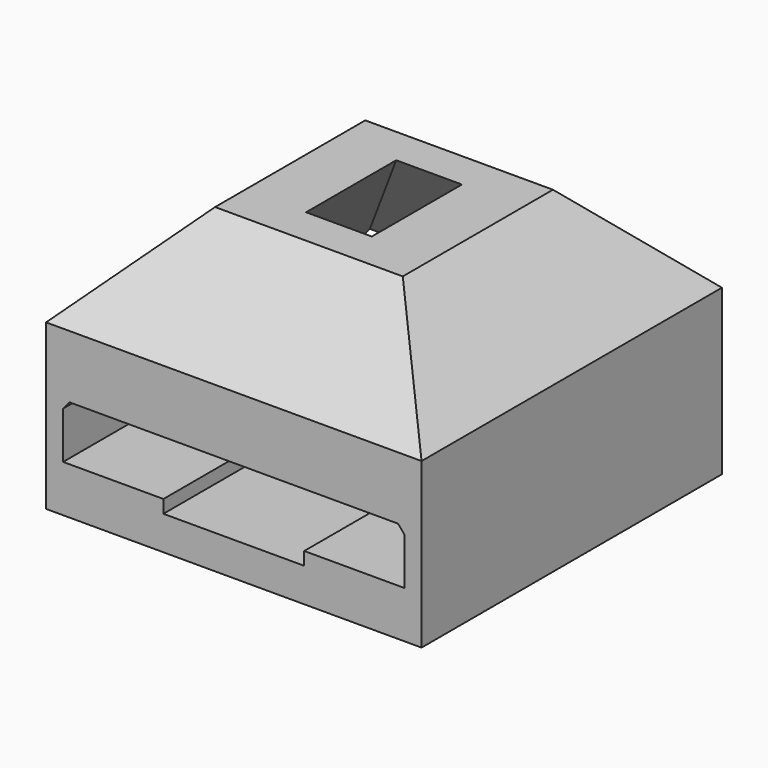
from build123d import *

# Parameters (mm, degrees)
F0_W     = 80
F0_H     = 80
F1_DEPTH = 55
F2_SIZE2 = 20
F2_SIZE  = 20
F3_W     = 14
F3_H     = 24
F4_DEPTH = 35
F4_TAPER = -40
F5_W     = 15
F5_H     = 2.5
F5_H_2   = 5.2806121111
F6_DEPTH = 50
F7_DEPTH = 10
F8_DEPTH = 5


# Not quite as in the source:
# - a feature names something its author has since deleted; it is built from what else it names


with BuildPart() as f1:
    # F0 (on Top) → F1 (new body)
    with BuildSketch(Plane.XY):
        with Locations((3.4524537623, -3.0448271871)):
            Rectangle(F0_W, F0_H)
    extrude(amount=F1_DEPTH)

    # F2
    f2_edges = [f1.edges().sort_by_distance(p)[0] for p in [
        (43.452454, -3.044827, 55),
        (3.452454, 36.955173, 55),
        (-36.547546, -3.044827, 55),
        (3.452454, -43.044827, 55),
    ]]
    chamfer(f2_edges, length=F2_SIZE, length2=F2_SIZE2)

    # F3 (on face) → F4 (cut)
    with BuildSketch(Plane.XY.offset(55)):
        with Locations((3.4524537623, -3.0448271871)):
            Rectangle(F3_W, F3_H)
    extrude(amount=-F4_DEPTH, taper=F4_TAPER, mode=Mode.SUBTRACT)

    # F5 (on face) → F6 (cut)
    with BuildSketch(Plane.XZ.offset(43.0448271871)):
        with Locations((10.9524537623, 18.75)):
            Rectangle(F5_W, F5_H)
        with Locations((-4.0475462377, 18.75)):
            Rectangle(F5_W, F5_H)
        with Locations((-4.0475462377, 14.8596939445)):
            Rectangle(F5_W, F5_H_2)
        with Locations((10.9524537623, 14.8596939445)):
            Rectangle(F5_W, F5_H_2)
    extrude(amount=-F6_DEPTH, mode=Mode.SUBTRACT)

    # F7 (cut): a face of the model
    f7_faces = [f1.faces().sort_by_distance(p)[0] for p in [
        (3.4524537623, 35.8739389153, 20),
    ]]
    extrude(f7_faces, amount=-F7_DEPTH, mode=Mode.SUBTRACT)

    # F8 (cut): a face of the model
    f8_faces = [f1.faces().sort_by_distance(p)[0] for p in [
        (3.4524537623, -18.0448271871, 12.2193878889),
    ]]
    extrude(f8_faces, amount=-F8_DEPTH, mode=Mode.SUBTRACT)


solid = f1.part
